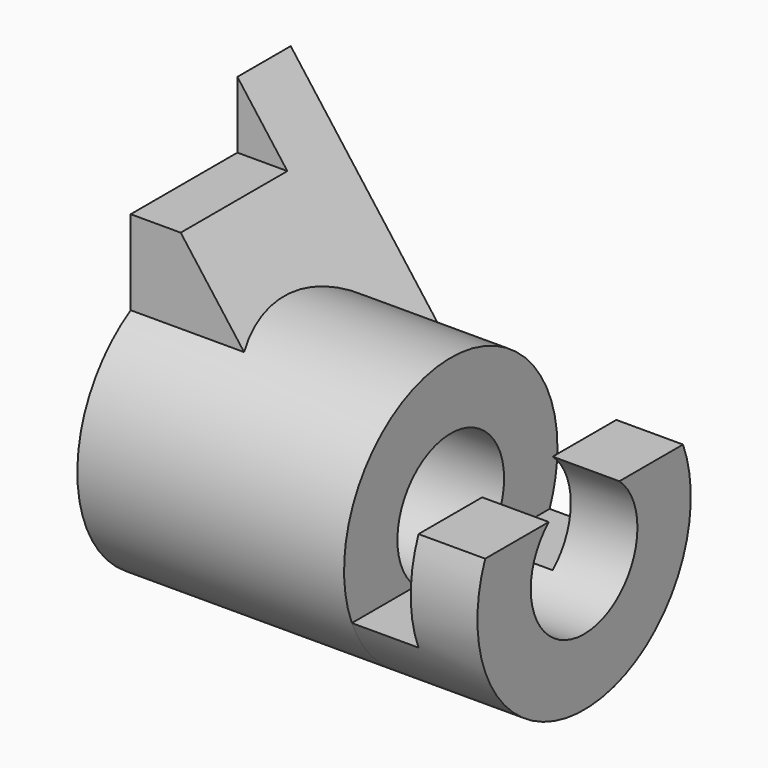
from build123d import *
from build123d import SkipClean  # not in build123d's __all__

# Parameters (mm, degrees)
F0_R      = 25.4
F0_R_2    = 12.7
F1_DEPTH  = 50.8
F3_DEPTH  = 12.7
F5_DEPTH  = 12.7
F8_DEPTH  = 25.4
F10_DEPTH = 12.7


# Not quite as in the source:
# - after a boolean that leaves OpenCascade's solid faulty, fix() repairs it


with BuildPart() as f1:
    # F0 (on Right) → F1 (new body)
    with BuildSketch(Plane.YZ):
        Circle(F0_R)
        Circle(F0_R_2, mode=Mode.SUBTRACT)
    extrude(amount=F1_DEPTH)

    # F2 (on face) → F3 (join)
    with BuildSketch(Plane.YZ.offset(50.8)):
        with BuildLine():
            Line((-8.4002604126, -9.525), (-23.5464301965, -9.525))
            ThreePointArc((-23.5464301965, -9.525), (0, -25.4), (23.5464301965, -9.525))
            Line((23.5464301965, -9.525), (8.4002604126, -9.525))
            ThreePointArc((8.4002604126, -9.525), (0, -12.7), (-8.4002604126, -9.525))
        make_face()
    extrude(amount=F3_DEPTH)

    # F4 (on face) → F5 (join)
    with BuildSketch(Plane.YZ.offset(63.5)):
        with BuildLine():
            ThreePointArc((-23.5464301965, -9.525), (0, -25.4), (23.5464301965, -9.525))
            ThreePointArc((23.5464301965, -9.525), (25.4, 0), (23.5464301965, 9.525))
            Line((23.5464301965, 9.525), (8.4002604126, 9.525))
            ThreePointArc((8.4002604126, 9.525), (12.7, 0), (8.4002604126, -9.525))
            ThreePointArc((8.4002604126, -9.525), (0, -12.7), (-8.4002604126, -9.525))
            ThreePointArc((-8.4002604126, -9.525), (-12.7, 0), (-8.4002604126, 9.525))
            Line((-8.4002604126, 9.525), (-23.5464301965, 9.525))
            ThreePointArc((-23.5464301965, 9.525), (-25.4, 0), (-23.5464301965, -9.525))
        make_face()
    with SkipClean():  # cleaning this boolean's faces spoils the solid; the shape is the same uncleaned
        extrude(amount=F5_DEPTH)

    # F7 (on offset) → F8 (join)
    with BuildSketch(Plane.XZ.offset(12.7)):
        Polygon((0, 38.1), (0, 25.4), (19.05, 25.4), (9.525, 38.1), align=None)
        Polygon((0, 25.4), (0, 19.05), (23.8125, 19.05), (19.05, 25.4), align=None)
    extrude(amount=-F8_DEPTH)

    add(f1.part.fix(), mode=Mode.REPLACE)

    # F9 (on face) → F10 (join)
    with BuildSketch(Plane(origin=(0, 12.7, 0), x_dir=(-1, 0, 0), z_dir=(0, 1, 0))):
        Polygon((-38.1, 0), (0, 0), (0, 50.8), (-19.05, 25.4), align=None)
    extrude(amount=F10_DEPTH)


solid = f1.part
